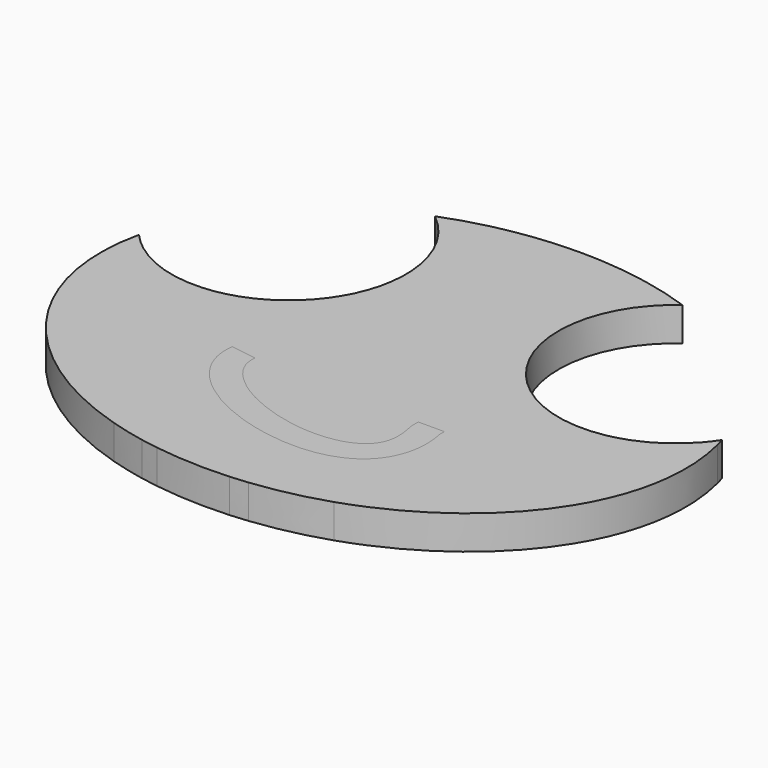
from build123d import *

# Parameters (mm, degrees)
F1_DEPTH = 5
F2_DEPTH = 5


with BuildPart() as f1:
    # F0 (on Top) → F1 (new body)
    with BuildSketch(Plane.XY):
        with BuildLine():
            add(Edge.make_bspline(
                [(12.734443, -39.781365), (15.920232, -37.835476), (17.632841, -33.879291), (16.61114, -28.898724)],
                knots=[0, 0, 0, 0, 1, 1, 1, 1], degree=3))
            Line((16.61114, -28.898724), (16.61114, -28.020637))
            Line((16.61114, -28.020637), (12.746019, -28.020637))
            add(Edge.make_bspline(
                [(12.746019, -28.020637), (12.746019, -28.0208513466), (12.746019, -28.0210702537), (12.746019, -28.0378303299), (12.746019, -28.3570972405), (12.746019, -28.6929007595), (12.746019, -29.0121676701), (12.746019, -29.0289277463), (12.746019, -29.0291466534), (12.746019, -29.029361)],
                knots=[0, 0, 0, 0, 0.0006430397, 0.0006567214, 0.0502802287, 0.9584437713, 1.0080672786, 1.0080809603, 1.008724, 1.008724, 1.008724, 1.008724], degree=3))
            add(Edge.make_bspline(
                [(12.746019, -29.029361), (12.74605, -29.172341), (12.761948, -29.314876), (12.793421, -29.454349)],
                knots=[0, 0, 0, 0, 1, 1, 1, 1], degree=3))
            add(Edge.make_bspline(
                [(12.793421, -29.454349), (13.710785, -33.520561), (12.70048, -35.27361), (10.719751, -36.483446)],
                knots=[0, 0, 0, 0, 1, 1, 1, 1], degree=3))
            add(Edge.make_bspline(
                [(10.719751, -36.483446), (8.739023, -37.693279), (5.281256, -38.058505), (1.640132, -37.446969)],
                knots=[0, 0, 0, 0, 1, 1, 1, 1], degree=3))
            add(Edge.make_bspline(
                [(1.640132, -37.446969), (-2.000989, -36.835433), (-5.782567, -35.302924), (-8.385923, -33.358605)],
                knots=[0, 0, 0, 0, 1, 1, 1, 1], degree=3))
            add(Edge.make_bspline(
                [(-8.385923, -33.358605), (-10.989276, -31.414286), (-12.239972, -29.310328), (-11.946774, -27.289724)],
                knots=[0, 0, 0, 0, 1, 1, 1, 1], degree=3))
            Line((-11.946774, -27.289724), (-15.771656, -26.734652))
            add(Edge.make_bspline(
                [(-15.771656, -26.734652), (-16.337542, -30.634506), (-13.932498, -34.039847), (-10.698271, -36.455334)],
                knots=[0, 0, 0, 0, 1, 1, 1, 1], degree=3))
            add(Edge.make_bspline(
                [(-10.698271, -36.455334), (-7.464044, -38.870817), (-3.226178, -40.548244), (1.00017, -41.25807)],
                knots=[0, 0, 0, 0, 1, 1, 1, 1], degree=3))
            add(Edge.make_bspline(
                [(1.00017, -41.25807), (5.226522, -41.967898), (9.484578, -41.766392), (12.734443, -39.781365)],
                knots=[0, 0, 0, 0, 1, 1, 1, 1], degree=3))
        make_face()
    extrude(amount=F1_DEPTH)


with BuildPart() as f1b:
    # F0 (on Top) → F1, piece 2 (new body)
    with BuildSketch(Plane.XY):
        with BuildLine():
            add(Edge.make_bspline(
                [(-27.7454914934, -17.3831615798), (-25.4848622372, -19.2736486235), (-23.4287961137, -21.451514347), (-21.6284719984, -23.9119219826)],
                knots=[0.8661202793, 0.8661202793, 0.8661202793, 0.8661202793, 1, 1, 1, 1], degree=3))
            add(Edge.make_bspline(
                [(-27.7454914981, -17.3831615977), (-28.0822081964, -17.4027131688), (-28.4214851444, -17.412626), (-28.76305, -17.412626)],
                knots=[0.9642809302, 0.9642809302, 0.9642809302, 0.9642809302, 1, 1, 1, 1], degree=3))
            add(Edge.make_bspline(
                [(-28.7630500014, -17.4126260018), (-33.8960829139, -17.4126260018), (-38.5015979977, -15.1739896926), (-41.6668967581, -11.6268322113)],
                knots=[0, 0, 0, 0, 0.5367857347, 0.5367857347, 0.5367857347, 0.5367857347], degree=3))
            add(Edge.make_bspline(
                [(-42.3593879972, -17.8232599981), (-42.3593879972, -15.70835477), (-42.1218509095, -13.6374762635), (-41.6668967569, -11.6268322116)],
                knots=[0, 0, 0, 0, 0.1108003269, 0.1108003269, 0.1108003269, 0.1108003269], degree=3))
            add(Edge.make_bspline(
                [(-14.5369517464, -50.1506168986), (-30.8120747848, -45.1875138054), (-42.359388, -32.5977476883), (-42.359388, -17.82326)],
                knots=[0.2274692045, 0.2274692045, 0.2274692045, 0.2274692045, 1, 1, 1, 1], degree=3))
            add(Edge.make_bspline(
                [(-21.628472002, -23.9119220042), (-15.9783217735, -31.6281219583), (-13.7253066716, -40.8854651209), (-14.5369517491, -50.1506168989)],
                knots=[0, 0, 0, 0, 0.4190171031, 0.4190171031, 0.4190171031, 0.4190171031], degree=3))
        make_face()
    extrude(amount=F1_DEPTH)



with BuildPart() as f1c:
    # F0 (on Top) → F1, piece 3 (new body)
    with BuildSketch(Plane.XY):
        with BuildLine():
            add(Edge.make_bspline(
                [(41.496607571, -11.5207741803), (39.0096189113, -14.3537933789), (35.6115250768, -16.3700235375), (31.7572682547, -17.1057755436)],
                knots=[0.457889602, 0.457889602, 0.457889602, 0.457889602, 0.8834983945, 0.8834983945, 0.8834983945, 0.8834983945], degree=3))
            add(Edge.make_bspline(
                [(24.801034, -24.322837), (26.8241254465, -21.5600342644), (29.1667116086, -19.1520336904), (31.7572682547, -17.1057755436)],
                knots=[0, 0, 0, 0, 0.1500300155, 0.1500300155, 0.1500300155, 0.1500300155], degree=3))
            add(Edge.make_bspline(
                [(17.6440274537, -49.729019344), (17.0311754569, -40.7368621909), (19.3145165012, -31.800141131), (24.801034, -24.322837)],
                knots=[0.593126466, 0.593126466, 0.593126466, 0.593126466, 1, 1, 1, 1], degree=3))
            add(Edge.make_bspline(
                [(44.149908, -17.82326), (44.149908, -32.1960737794), (33.2217734232, -44.5013432134), (17.6440274514, -49.7290193437)],
                knots=[0, 0, 0, 0, 0.7515280054, 0.7515280054, 0.7515280054, 0.7515280054], degree=3))
            add(Edge.make_bspline(
                [(43.2741469204, -10.8659114346), (43.8483964355, -13.1136924153), (44.149908, -15.4405345256), (44.149908, -17.82326)],
                knots=[0.8751685145, 0.8751685145, 0.8751685145, 0.8751685145, 1, 1, 1, 1], degree=3))
            add(Edge.make_bspline(
                [(41.496607571, -11.5207741803), (42.0831921323, -11.2889186769), (42.6758725904, -11.0706148581), (43.2741469213, -10.8659114372)],
                knots=[0.3213713892, 0.3213713892, 0.3213713892, 0.3213713892, 0.3500969523, 0.3500969523, 0.3500969523, 0.3500969523], degree=3))
        make_face()
        with BuildLine():
            add(Edge.make_bspline(
                [(42.9322474575, -9.6419037564), (42.4962572948, -10.3010425075), (42.0163267182, -10.9287432049), (41.496607571, -11.5207741803)],
                knots=[0.3689478861, 0.3689478861, 0.3689478861, 0.3689478861, 0.457889602, 0.457889602, 0.457889602, 0.457889602], degree=3))
            add(Edge.make_bspline(
                [(41.496607571, -11.5207741803), (42.0831921323, -11.2889186769), (42.6758725904, -11.0706148581), (43.2741469213, -10.8659114372)],
                knots=[0.3213713892, 0.3213713892, 0.3213713892, 0.3213713892, 0.3500969523, 0.3500969523, 0.3500969523, 0.3500969523], degree=3))
            add(Edge.make_bspline(
                [(42.9322474577, -9.6419037563), (43.0552016039, -10.0471728179), (43.1692265907, -10.4552224997), (43.2741469204, -10.8659114346)],
                knots=[0.8523607274, 0.8523607274, 0.8523607274, 0.8523607274, 0.8751685145, 0.8751685145, 0.8751685145, 0.8751685145], degree=3))
        make_face()
    extrude(amount=F1_DEPTH)


with BuildPart() as f1b_1:
    add(f1b.part)

    add(f1c.part)  # F2 merges F1c
    # F0 (on Top) → F2 (join)
    with BuildSketch(Plane.XY):
        with BuildLine():
            add(Edge.make_bspline(
                [(-5.9378795005, 16.3365863681), (-4.9497466604, 16.4619585653), (-3.9504295333, 16.560578393), (-2.9411196849, 16.6314859824)],
                knots=[0.9027302545, 0.9027302545, 0.9027302545, 0.9027302545, 0.9459190297, 0.9459190297, 0.9459190297, 0.9459190297], degree=3))
            add(Edge.make_bspline(
                [(-17.8832007592, 13.3451160525), (-14.1667628508, 14.7796245747), (-10.1541337023, 15.8016369849), (-5.9378795005, 16.3365863681)],
                knots=[0.7184484983, 0.7184484983, 0.7184484983, 0.7184484983, 0.9027302545, 0.9027302545, 0.9027302545, 0.9027302545], degree=3))
            add(Edge.make_bspline(
                [(-17.8832007591, 13.3451160522), (-13.9495167672, 10.1766095439), (-11.431219, 5.3257917383), (-11.431219, -0.118331)],
                knots=[0.4306821184, 0.4306821184, 0.4306821184, 0.4306821184, 1, 1, 1, 1], degree=3))
            add(Edge.make_bspline(
                [(-11.431219, -0.118331), (-11.431219, -9.3028339682), (-18.6554034185, -16.855342504), (-27.7454914981, -17.3831615977)],
                knots=[0, 0, 0, 0, 0.9642809302, 0.9642809302, 0.9642809302, 0.9642809302], degree=3))
            add(Edge.make_bspline(
                [(-27.7454914934, -17.3831615798), (-25.4848622372, -19.2736486235), (-23.4287961137, -21.451514347), (-21.6284719984, -23.9119219826)],
                knots=[0.8661202793, 0.8661202793, 0.8661202793, 0.8661202793, 1, 1, 1, 1], degree=3))
            add(Edge.make_bspline(
                [(-21.628472002, -23.9119220042), (-15.9783217735, -31.6281219583), (-13.7253066716, -40.8854651209), (-14.5369517491, -50.1506168989)],
                knots=[0, 0, 0, 0, 0.4190171031, 0.4190171031, 0.4190171031, 0.4190171031], degree=3))
            add(Edge.make_bspline(
                [(-9.358816, -51.4367196264), (-11.1301489273, -51.0930942082), (-12.8586867056, -50.6624042685), (-14.5369517464, -50.1506168986)],
                knots=[0.1478070462, 0.1478070462, 0.1478070462, 0.1478070462, 0.2274692045, 0.2274692045, 0.2274692045, 0.2274692045], degree=3))
            add(Edge.make_bspline(
                [(-6.77968, -51.8706532523), (-7.6486983636, -51.7465029707), (-8.5086859107, -51.6016385431), (-9.358816, -51.4367196264)],
                knots=[0.1095741445, 0.1095741445, 0.1095741445, 0.1095741445, 0.1478070462, 0.1478070462, 0.1478070462, 0.1478070462], degree=3))
            add(Edge.make_bspline(
                [(0.895119, -52.412133), (-1.7243512939, -52.412133), (-4.2891040964, -52.2264635695), (-6.77968, -51.8706532523)],
                knots=[0, 0, 0, 0, 0.1095741445, 0.1095741445, 0.1095741445, 0.1095741445], degree=3))
            add(Edge.make_bspline(
                [(4.274391, -52.3084107676), (3.1593420107, -52.3771353208), (2.032387159, -52.412133), (0.895119, -52.412133)],
                knots=[0.9524273319, 0.9524273319, 0.9524273319, 0.9524273319, 1, 1, 1, 1], degree=3))
            add(Edge.make_bspline(
                [(6.8688456197, -52.0857892042), (6.0118230737, -52.1802340142), (5.1467506657, -52.2546440462), (4.274391, -52.3084107676)],
                knots=[0.9152088086, 0.9152088086, 0.9152088086, 0.9152088086, 0.9524273319, 0.9524273319, 0.9524273319, 0.9524273319], degree=3))
            add(Edge.make_bspline(
                [(17.6440274514, -49.7290193437), (14.2512357594, -50.8675933181), (10.6378865758, -51.670436821), (6.8688456197, -52.0857892042)],
                knots=[0.7515280054, 0.7515280054, 0.7515280054, 0.7515280054, 0.9152088086, 0.9152088086, 0.9152088086, 0.9152088086], degree=3))
            add(Edge.make_bspline(
                [(17.6440274537, -49.729019344), (17.0311754569, -40.7368621909), (19.3145165012, -31.800141131), (24.801034, -24.322837)],
                knots=[0.593126466, 0.593126466, 0.593126466, 0.593126466, 1, 1, 1, 1], degree=3))
            add(Edge.make_bspline(
                [(24.801034, -24.322837), (26.8241254465, -21.5600342644), (29.1667116086, -19.1520336904), (31.7572682547, -17.1057755436)],
                knots=[0, 0, 0, 0, 0.1500300155, 0.1500300155, 0.1500300155, 0.1500300155], degree=3))
            add(Edge.make_bspline(
                [(31.7572682547, -17.1057755436), (30.7022451548, -17.30717244), (29.6130427928, -17.4126260015), (28.4989919964, -17.4126260015)],
                knots=[0.8834983945, 0.8834983945, 0.8834983945, 0.8834983945, 1, 1, 1, 1], degree=3))
            add(Edge.make_bspline(
                [(28.498992, -17.412626), (18.936739, -17.412626), (11.167443, -9.643331), (11.167443, -0.118331)],
                knots=[0, 0, 0, 0, 1, 1, 1, 1], degree=3))
            add(Edge.make_bspline(
                [(11.1674430006, -0.1183309997), (11.1674430006, 5.627639161), (13.9726326914, 10.7126893493), (18.2864119041, 13.856445722)],
                knots=[0, 0, 0, 0, 0.6008835063, 0.6008835063, 0.6008835063, 0.6008835063], degree=3))
            add(Edge.make_bspline(
                [(7.5071641473, 16.3641522212), (11.2838455632, 15.9010039293), (14.8989934452, 15.0473276915), (18.2864119041, 13.8564457219)],
                knots=[0.0940532477, 0.0940532477, 0.0940532477, 0.0940532477, 0.25884533, 0.25884533, 0.25884533, 0.25884533], degree=3))
            add(Edge.make_bspline(
                [(4.5089480455, 16.6466515848), (5.5186328345, 16.5798891894), (6.5184341258, 16.4854038096), (7.5071641473, 16.3641522212)],
                knots=[0.0509109063, 0.0509109063, 0.0509109063, 0.0509109063, 0.0940532477, 0.0940532477, 0.0940532477, 0.0940532477], degree=3))
            add(Edge.make_bspline(
                [(0.895119, 16.765614), (2.112190798, 16.765614), (3.3174511085, 16.7254357662), (4.5089480455, 16.6466515848)],
                knots=[0, 0, 0, 0, 0.0509109063, 0.0509109063, 0.0509109063, 0.0509109063], degree=3))
            add(Edge.make_bspline(
                [(-2.9411196849, 16.6314859824), (-1.6772622212, 16.7202764427), (-0.3977361304, 16.7656140019), (0.8951190028, 16.7656140019)],
                knots=[0.9459190297, 0.9459190297, 0.9459190297, 0.9459190297, 1, 1, 1, 1], degree=3))
        make_face()
        with BuildLine():
            Line((16.61114, -28.020637), (16.61114, -28.898724))
            add(Edge.make_bspline(
                [(12.734443, -39.781365), (15.920232, -37.835476), (17.632841, -33.879291), (16.61114, -28.898724)],
                knots=[0, 0, 0, 0, 1, 1, 1, 1], degree=3))
            add(Edge.make_bspline(
                [(1.00017, -41.25807), (5.226522, -41.967898), (9.484578, -41.766392), (12.734443, -39.781365)],
                knots=[0, 0, 0, 0, 1, 1, 1, 1], degree=3))
            add(Edge.make_bspline(
                [(-10.698271, -36.455334), (-7.464044, -38.870817), (-3.226178, -40.548244), (1.00017, -41.25807)],
                knots=[0, 0, 0, 0, 1, 1, 1, 1], degree=3))
            add(Edge.make_bspline(
                [(-15.771656, -26.734652), (-16.337542, -30.634506), (-13.932498, -34.039847), (-10.698271, -36.455334)],
                knots=[0, 0, 0, 0, 1, 1, 1, 1], degree=3))
            Line((-15.771656, -26.734652), (-11.946774, -27.289724))
            add(Edge.make_bspline(
                [(-8.385923, -33.358605), (-10.989276, -31.414286), (-12.239972, -29.310328), (-11.946774, -27.289724)],
                knots=[0, 0, 0, 0, 1, 1, 1, 1], degree=3))
            add(Edge.make_bspline(
                [(1.640132, -37.446969), (-2.000989, -36.835433), (-5.782567, -35.302924), (-8.385923, -33.358605)],
                knots=[0, 0, 0, 0, 1, 1, 1, 1], degree=3))
            add(Edge.make_bspline(
                [(10.719751, -36.483446), (8.739023, -37.693279), (5.281256, -38.058505), (1.640132, -37.446969)],
                knots=[0, 0, 0, 0, 1, 1, 1, 1], degree=3))
            add(Edge.make_bspline(
                [(12.793421, -29.454349), (13.710785, -33.520561), (12.70048, -35.27361), (10.719751, -36.483446)],
                knots=[0, 0, 0, 0, 1, 1, 1, 1], degree=3))
            add(Edge.make_bspline(
                [(12.746019, -29.029361), (12.74605, -29.172341), (12.761948, -29.314876), (12.793421, -29.454349)],
                knots=[0, 0, 0, 0, 1, 1, 1, 1], degree=3))
            add(Edge.make_bspline(
                [(12.746019, -28.020637), (12.746019, -28.0208513466), (12.746019, -28.0210702537), (12.746019, -28.0378303299), (12.746019, -28.3570972405), (12.746019, -28.6929007595), (12.746019, -29.0121676701), (12.746019, -29.0289277463), (12.746019, -29.0291466534), (12.746019, -29.029361)],
                knots=[0, 0, 0, 0, 0.0006430397, 0.0006567214, 0.0502802287, 0.9584437713, 1.0080672786, 1.0080809603, 1.008724, 1.008724, 1.008724, 1.008724], degree=3))
            Line((12.746019, -28.020637), (16.61114, -28.020637))
        make_face(mode=Mode.SUBTRACT)
    extrude(amount=F2_DEPTH)


solid = Compound([f1.part, f1b_1.part])
